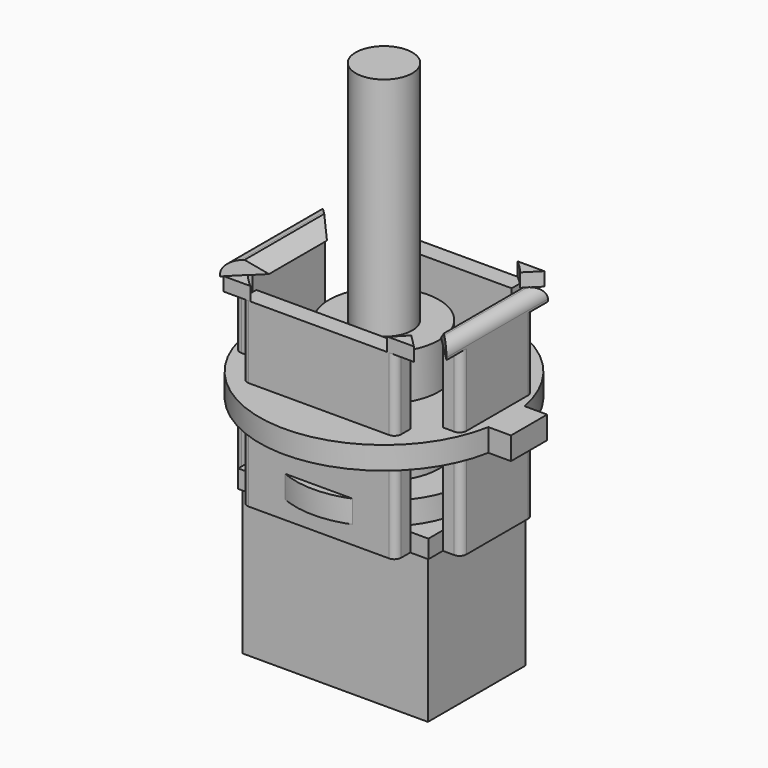
from build123d import *

# Parameters (mm, degrees)
F2_R           = 2.425
F2_R_2         = 1.25
F3_DEPTH       = 7.2
F4_DEPTH       = 6
F5_DEPTH       = 1
F6_START       = 3
F6_DEPTH       = 1
F7_DEPTH       = 16
F8_W           = 6.8
F8_H           = 0.8
F8_W_2         = 0.8
F8_H_2         = 4
F9_DEPTH       = 0.8
F10_DEPTH      = 7.2
F10_DEPTH_BACK = 0.8
F12_DEPTH      = 0.6
F13_R          = 0.5
F14_R          = 0.3
F15_T4_DEPTH   = 7.5433659759
F15_T10_DEPTH  = 7.5433659759


# Not quite as in the source:
# - a fillet or chamfer that OpenCascade refuses, or shapes differently, is made with other operations: its cross-section is extruded or revolved along the edge and cut away or added
# - a feature names something its author has since deleted; it is built from what else it names


with BuildPart() as f3:
    # F2 (on Top) → F3 (new body)
    with BuildSketch(Plane.XY):
        with BuildLine():
            Line((-2.8142494559, -2.7), (2.8142494559, -2.7))
            ThreePointArc((2.8142494559, -2.7), (3.6183955614, -1.4550647962), (3.9, 0))
            ThreePointArc((3.9, 0), (3.6183955614, 1.4550647962), (2.8142494559, 2.7))
            Line((2.8142494559, 2.7), (-2.8142494559, 2.7))
            ThreePointArc((-2.8142494559, 2.7), (-3.9, 0), (-2.8142494559, -2.7))
        make_face()
        Circle(F2_R, mode=Mode.SUBTRACT)
        Circle(F2_R)
        Circle(F2_R_2, mode=Mode.SUBTRACT)
        Circle(F2_R_2)
        with BuildLine():
            Line((2.8142494559, -2.7), (4.1, -2.7))
            Line((4.1, -2.7), (4.1, 2.7))
            Line((4.1, 2.7), (2.8142494559, 2.7))
            ThreePointArc((2.8142494559, 2.7), (3.6183955614, 1.4550647962), (3.9, 0))
            ThreePointArc((3.9, 0), (3.6183955614, -1.4550647962), (2.8142494559, -2.7))
        make_face()
        with BuildLine():
            Line((-4.1, -2.7), (-2.8142494559, -2.7))
            ThreePointArc((-2.8142494559, -2.7), (-3.9, 0), (-2.8142494559, 2.7))
            Line((-2.8142494559, 2.7), (-4.1, 2.7))
            Line((-4.1, 2.7), (-4.1, -2.7))
        make_face()
    extrude(amount=-F3_DEPTH)

    # F2 (on Top) → F4 (join)
    with BuildSketch(Plane.XY):
        Circle(F2_R)
        Circle(F2_R_2, mode=Mode.SUBTRACT)
        Circle(F2_R_2)
    extrude(amount=F4_DEPTH)

    # F2 (on Top) → F7 (join)
    with BuildSketch(Plane.XY):
        Circle(F2_R_2)
    extrude(amount=F7_DEPTH)


with BuildPart() as f5:
    # F2 (on Top) → F5 (new body)
    with BuildSketch(Plane.XY):
        with BuildLine():
            Line((-2.8142494559, -2.7), (2.8142494559, -2.7))
            ThreePointArc((2.8142494559, -2.7), (3.6183955614, -1.4550647962), (3.9, 0))
            ThreePointArc((3.9, 0), (3.6183955614, 1.4550647962), (2.8142494559, 2.7))
            Line((2.8142494559, 2.7), (-2.8142494559, 2.7))
            ThreePointArc((-2.8142494559, 2.7), (-3.9, 0), (-2.8142494559, -2.7))
        make_face()
        Circle(F2_R, mode=Mode.SUBTRACT)
        with BuildLine():
            ThreePointArc((-2.8142494559, -2.7), (0, -3.9), (2.8142494559, -2.7))
            Line((2.8142494559, -2.7), (-2.8142494559, -2.7))
        make_face()
        with BuildLine():
            Line((-2.8142494559, 2.7), (2.8142494559, 2.7))
            ThreePointArc((2.8142494559, 2.7), (0, 3.9), (-2.8142494559, 2.7))
        make_face()
    extrude(amount=F5_DEPTH)


with BuildPart() as f6:
    # F2 (on Top) → F6 (new body)
    with BuildSketch(Plane.XY.offset(F6_START)):
        with BuildLine():
            Line((5.4083269132, -1), (5.4083269132, 1))
            ThreePointArc((5.4083269132, 1), (-5.5, 0), (5.4083269132, -1))
        make_face()
        with BuildLine():
            Line((4.1, 2.7), (4.1, -2.7))
            Line((4.1, -2.7), (2.8142494559, -2.7))
            ThreePointArc((2.8142494559, -2.7), (0, -3.9), (-2.8142494559, -2.7))
            Line((-2.8142494559, -2.7), (-4.1, -2.7))
            Line((-4.1, -2.7), (-4.1, 2.7))
            Line((-4.1, 2.7), (-2.8142494559, 2.7))
            ThreePointArc((-2.8142494559, 2.7), (0, 3.9), (2.8142494559, 2.7))
            Line((2.8142494559, 2.7), (4.1, 2.7))
        make_face(mode=Mode.SUBTRACT)
        with BuildLine():
            Line((-4.1, -2.7), (-2.8142494559, -2.7))
            ThreePointArc((-2.8142494559, -2.7), (-3.9, 0), (-2.8142494559, 2.7))
            Line((-2.8142494559, 2.7), (-4.1, 2.7))
            Line((-4.1, 2.7), (-4.1, -2.7))
        make_face()
        with BuildLine():
            Line((2.8142494559, -2.7), (4.1, -2.7))
            Line((4.1, -2.7), (4.1, 2.7))
            Line((4.1, 2.7), (2.8142494559, 2.7))
            ThreePointArc((2.8142494559, 2.7), (3.6183955614, 1.4550647962), (3.9, 0))
            ThreePointArc((3.9, 0), (3.6183955614, -1.4550647962), (2.8142494559, -2.7))
        make_face()
        with BuildLine():
            ThreePointArc((5.4083269132, 1), (5.4770337785, 0.502096593), (5.5, 0))
            ThreePointArc((5.5, 0), (5.4770337785, -0.502096593), (5.4083269132, -1))
            Line((5.4083269132, -1), (6.4083269132, -1))
            Line((6.4083269132, -1), (6.4083269132, 1))
            Line((6.4083269132, 1), (5.4083269132, 1))
        make_face()
        with BuildLine():
            ThreePointArc((5.4083269132, -1), (5.4770337785, -0.502096593), (5.5, 0))
            ThreePointArc((5.5, 0), (5.4770337785, 0.502096593), (5.4083269132, 1))
            Line((5.4083269132, 1), (5.4083269132, -1))
        make_face()
        with BuildLine():
            Line((-2.8142494559, 2.7), (2.8142494559, 2.7))
            ThreePointArc((2.8142494559, 2.7), (0, 3.9), (-2.8142494559, 2.7))
        make_face()
        with BuildLine():
            Line((-2.8142494559, -2.7), (2.8142494559, -2.7))
            ThreePointArc((2.8142494559, -2.7), (3.6183955614, -1.4550647962), (3.9, 0))
            ThreePointArc((3.9, 0), (3.6183955614, 1.4550647962), (2.8142494559, 2.7))
            Line((2.8142494559, 2.7), (-2.8142494559, 2.7))
            ThreePointArc((-2.8142494559, 2.7), (-3.9, 0), (-2.8142494559, -2.7))
        make_face()
        Circle(F2_R, mode=Mode.SUBTRACT)
        with BuildLine():
            ThreePointArc((-2.8142494559, -2.7), (0, -3.9), (2.8142494559, -2.7))
            Line((2.8142494559, -2.7), (-2.8142494559, -2.7))
        make_face()
    extrude(amount=F6_DEPTH)


with BuildPart() as f9:
    # F8 (on Top) → F9 (new body)
    with BuildSketch(Plane.XY):
        with Locations((0, 2.4)):
            Rectangle(F8_W, F8_H)
        with Locations((-3.8, 2.4)):
            Rectangle(F8_W_2, F8_H)
        with Locations((-3.8, 0)):
            Rectangle(F8_W_2, F8_H_2)
        with Locations((-3.8, -2.4)):
            Rectangle(F8_W_2, F8_H)
        with Locations((0, -2.4)):
            Rectangle(F8_W, F8_H)
        with Locations((3.8, 0)):
            Rectangle(F8_W_2, F8_H_2)
        with Locations((3.8, -2.4)):
            Rectangle(F8_W_2, F8_H)
        with Locations((3.8, 2.4)):
            Rectangle(F8_W_2, F8_H)
        with Locations((-4.6, 0)):
            Rectangle(F8_W_2, F8_H_2)
        with Locations((0, 3.2)):
            Rectangle(F8_W, F8_H)
        with Locations((0, -3.2)):
            Rectangle(F8_W, F8_H)
        with Locations((4.6, 0)):
            Rectangle(F8_W_2, F8_H_2)
    extrude(amount=-F9_DEPTH)

    # F8 (on Top) → F10 (join, two sides)
    with BuildSketch(Plane.XY) as f10_sk:
        with Locations((-4.6, 0)):
            Rectangle(F8_W_2, F8_H_2)
        with Locations((4.6, 0)):
            Rectangle(F8_W_2, F8_H_2)
        with Locations((0, -3.2)):
            Rectangle(F8_W, F8_H)
        with Locations((0, 3.2)):
            Rectangle(F8_W, F8_H)
    extrude(amount=F10_DEPTH)
    extrude(f10_sk.sketch, amount=-F10_DEPTH_BACK)

    # F11 (on face) → F12 (join)
    with BuildSketch(Plane.XY.offset(7.2)):
        with BuildLine():
            Line((-4.2360803561, 2.0360803561), (-5, 2.8))
            Line((-5, 2.8), (-5, -2.8))
            Line((-5, -2.8), (-4.2360803561, -2.0360803561))
            ThreePointArc((-4.2360803561, -2.0360803561), (-4.7, 0), (-4.2360803561, 2.0360803561))
        make_face()
        with BuildLine():
            Line((5, 2.8), (4.2360803561, 2.0360803561))
            ThreePointArc((4.2360803561, 2.0360803561), (4.2446955459, 2.0180584042), (4.2532340636, 2))
            Line((4.2532340636, 2), (5, 2))
            Line((5, 2), (5, 2.8))
        make_face()
        with BuildLine():
            Line((5, -2.8), (5, -2))
            Line((5, -2), (4.2532340636, -2))
            ThreePointArc((4.2532340636, -2), (4.2446955459, -2.0180584042), (4.2360803561, -2.0360803561))
            Line((4.2360803561, -2.0360803561), (5, -2.8))
        make_face()
        with BuildLine():
            Line((5, 2), (4.2532340636, 2))
            ThreePointArc((4.2532340636, 2), (4.5869488824, 1.0246462563), (4.7, 0))
            ThreePointArc((4.7, 0), (4.5869488824, -1.0246462563), (4.2532340636, -2))
            Line((4.2532340636, -2), (5, -2))
            Line((5, -2), (5, 2))
        make_face()
        with BuildLine():
            ThreePointArc((4.7, 0), (4.5869488824, 1.0246462563), (4.2532340636, 2))
            Line((4.2532340636, 2), (4.2, 2))
            Line((4.2, 2), (4.2, -2))
            Line((4.2, -2), (4.2532340636, -2))
            ThreePointArc((4.2532340636, -2), (4.5869488824, -1.0246462563), (4.7, 0))
        make_face()
        with BuildLine():
            Line((-3.0215889859, 3.6), (-4.2, 3.6))
            Line((-4.2, 3.6), (-3.6098338327, 3.0098338327))
            ThreePointArc((-3.6098338327, 3.0098338327), (-3.3288160322, 3.3179788763), (-3.0215889859, 3.6))
        make_face()
        with BuildLine():
            ThreePointArc((3.6098338327, -3.0098338327), (3.3288160322, -3.3179788763), (3.0215889859, -3.6))
            Line((3.0215889859, -3.6), (4.2, -3.6))
            Line((4.2, -3.6), (3.6098338327, -3.0098338327))
        make_face()
        with BuildLine():
            Line((4.2, 3.6), (3.0215889859, 3.6))
            ThreePointArc((3.0215889859, 3.6), (3.3288160322, 3.3179788763), (3.6098338327, 3.0098338327))
            Line((3.6098338327, 3.0098338327), (4.2, 3.6))
        make_face()
        with BuildLine():
            Line((-3.6098338327, -3.0098338327), (-4.2, -3.6))
            Line((-4.2, -3.6), (-3.0215889859, -3.6))
            ThreePointArc((-3.0215889859, -3.6), (-3.3288160322, -3.3179788763), (-3.6098338327, -3.0098338327))
        make_face()
        with BuildLine():
            Line((4.2532340636, -2), (4.2, -2))
            Line((4.2, -2), (4.2360803561, -2.0360803561))
            ThreePointArc((4.2360803561, -2.0360803561), (4.2446955459, -2.0180584042), (4.2532340636, -2))
        make_face()
        with BuildLine():
            ThreePointArc((4.2532340636, 2), (4.2446955459, 2.0180584042), (4.2360803561, 2.0360803561))
            Line((4.2360803561, 2.0360803561), (4.2, 2))
            Line((4.2, 2), (4.2532340636, 2))
        make_face()
        with BuildLine():
            Line((-3.4, 1.2), (-4.2360803561, 2.0360803561))
            ThreePointArc((-4.2360803561, 2.0360803561), (-4.7, 0), (-4.2360803561, -2.0360803561))
            Line((-4.2360803561, -2.0360803561), (-3.4, -1.2))
            Line((-3.4, -1.2), (-3.4, 1.2))
        make_face()
        Polygon((4.2, -2), (4.2, 2), (3.4, 1.2), (3.4, -1.2), align=None)
    extrude(amount=F12_DEPTH)

    # F13
    f13_edges = [f9.edges().sort_by_distance(p)[0] for p in [
        (-5, 0, 7.8),
        (5, 0, 7.8),
    ]]
    fillet(f13_edges, radius=F13_R)

    # F14
    f14_edges = [f9.edges().sort_by_distance(p)[0] for p in [
        (5, 2, 3.2),
        (3.4, 3.6, 3.2),
        (-3.4, 3.6, 3.2),
        (5, -2, 3.2),
        (3.4, -3.6, 3.2),
        (-3.4, -3.6, 3.2),
        (-5, -2, 3.2),
    ]]
    fillet(f14_edges, radius=F14_R)

    # F15: chamfer of 1 on 2 edges, made by hand


with BuildPart() as f15_tool2:
    # F15_s3 → F15_t4 (new body)
    with BuildSketch(Plane.XZ.offset(-3.771682988)):
        Polygon((4.4, 7.8), (3.4, 6.8), (3.4, 7.8), align=None)
    extrude(amount=F15_T4_DEPTH)

    split(bisect_by=Plane(origin=(1.1, -1.1, 0), x_dir=(0, 0, 1), z_dir=(0.7071067812, -0.7071067812, 0)), keep=Keep.TOP)

    split(bisect_by=Plane(origin=(0.3, 0.3, 0), x_dir=(0, 0, 1), z_dir=(0.7071067812, 0.7071067812, 0)), keep=Keep.TOP)


with BuildPart() as f9_1:
    add(f9.part)

    # F15_t1: cut F15_tool2
    add(f15_tool2.part, mode=Mode.SUBTRACT)


with BuildPart() as f15_tool8:
    # F15_s9 → F15_t10 (new body)
    with BuildSketch(Plane.XZ.offset(3.771682988)):
        Polygon((-4.4, 7.8), (-3.4, 6.8), (-3.4, 7.8), align=None)
    extrude(amount=-F15_T10_DEPTH)

    split(bisect_by=Plane.XZ.offset(-2.8), keep=Keep.TOP)

    split(bisect_by=Plane(origin=(-0.3, 0.3, 0), x_dir=(0, 0, 1), z_dir=(-0.7071067812, 0.7071067812, 0)), keep=Keep.TOP)


with BuildPart() as f9_2:
    add(f9_1.part)

    # F15_t7: cut F15_tool8
    add(f15_tool8.part, mode=Mode.SUBTRACT)


solid = Compound([f3.part, f5.part, f6.part, f9_2.part])
